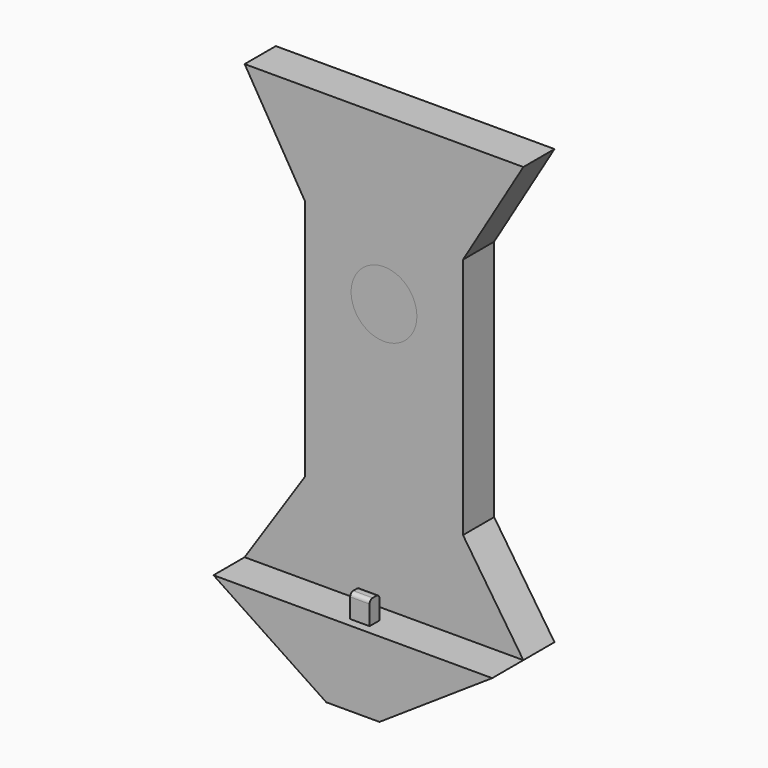
from build123d import *

# Parameters (mm, degrees)
F0_R     = 4.2213718129
F1_DEPTH = 5
F2_DEPTH = 10
F3_DEPTH = 2
F4_R     = 1.99999
F5_DEPTH = 5
F6_W     = 2.4935528636
F6_H     = 1.5890598297
F7_DEPTH = 3
F8_R     = 0.5


# Not quite as in the source:
# - a fillet or chamfer is up to 0.001 mm smaller than in the source, because OpenCascade refuses the exact size


with BuildPart() as f1:
    # F0 (on Front) → F1 (new body)
    with BuildSketch(Plane.XZ):
        Polygon((-17.8985148668, -23.0509787798), (17.8985148668, -23.0509787798), (10.1462722469, -11.4283849092), (10.1462722469, 19.7144318372), (17.8985148668, 32.7110886574), (-17.8985148668, 32.7110886574), (-10.1462722469, 19.7144318372), (-10.1462722469, -11.4283849092), align=None)
        with Locations((0, 11.391043663)):
            Circle(F0_R, mode=Mode.SUBTRACT)
    extrude(amount=F1_DEPTH)

    # F0 (on Front) → F2 (join)
    with BuildSketch(Plane.XZ):
        Polygon((-3.4155401514, -32.7110886574), (3.4155401514, -32.7110886574), (17.8985148668, -23.0509787798), (-17.8985148668, -23.0509787798), align=None)
    extrude(amount=F2_DEPTH)

    # F6 (on face) → F7 (join)
    with BuildSketch(Plane.XY.offset(-23.0509787798)):
        with Locations((0, -8.0799311399)):
            Rectangle(F6_W, F6_H)
    extrude(amount=F7_DEPTH)

    # F8
    f8_edges = [f1.edges().sort_by_distance(p)[0] for p in [
        (0, -8.874461, -20.050979),
        (0, -7.285401, -20.050979),
    ]]
    fillet(f8_edges, radius=F8_R)


with BuildPart() as f3:
    # F0 (on Front) → F3 (new body)
    with BuildSketch(Plane.XZ):
        with Locations((0, 11.391043663)):
            Circle(F0_R)
    extrude(amount=-F3_DEPTH)

    # F4 (radius 2 in the source; OpenCascade refuses exactly that, so slightly less here)
    f4_edges = [f3.edges().sort_by_distance(p)[0] for p in [
        (-4.221372, 2, 11.391044),
    ]]
    fillet(f4_edges, radius=F4_R)


with BuildPart() as f5:
    # F0 (on Front) → F5 (new body)
    with BuildSketch(Plane.XZ):
        with Locations((0, 11.391043663)):
            Circle(F0_R)
    extrude(amount=F5_DEPTH)


solid = Compound([f1.part, f3.part, f5.part])
